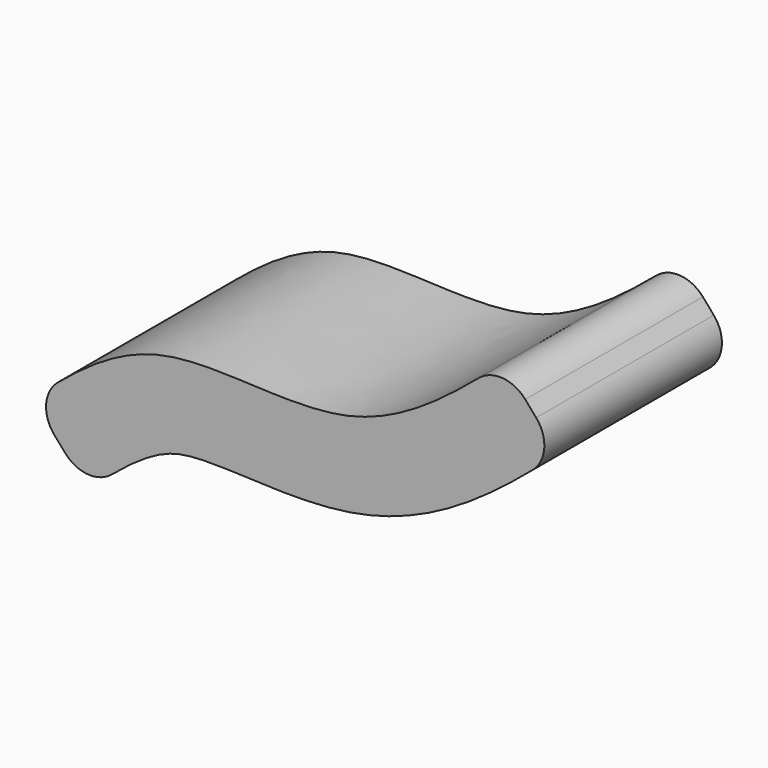
from build123d import *

# Parameters (mm, degrees)
F1_DEPTH = 50.8
F2_R     = 7.62


# Not quite as in the source:
# - the dataset's text gives a spline's control points without its knots; the knots are read off the source's solid


with BuildPart() as f1:
    # F0 (on Front) → F1 (new body)
    with BuildSketch(Plane.XZ):
        with BuildLine():
            add(Edge.make_bspline(
                [(-46.1671091616, 0), (-37.1033304025, 7.9272261416), (-18.0786162948, 24.5663360559), (28.0755181864, 12.987372443), (50.4588119298, 32.4166765689), (61.6594180465, 42.1391054988)],
                knots=[0, 0, 0, 0, 0.3125267415, 0.6559881994, 1, 1, 1, 1], degree=3))
            Line((-46.1671091616, 0), (-33.6258047307, -14.3393927058))
            add(Edge.make_bspline(
                [(-33.6258047307, -14.3393927058), (-31.8132040881, -12.7540831368), (-29.2307453089, -10.4982277646), (-26.0239095445, -7.8573374421), (-23.7368914894, -6.0858011695), (-21.5707475447, -4.5442227641), (-19.5307469779, -3.245218017), (-17.9388050177, -2.3665345235), (-16.727470375, -1.7805087063), (-15.8478404371, -1.3968942034), (-14.9938941443, -1.0662973184), (-14.1605211756, -0.7853779615), (-13.4786898496, -0.5901216464), (-12.9347342127, -0.4553712905), (-12.5313477685, -0.3657981044), (-12.1108276326, -0.2832227824), (-11.499360182, -0.1779155125), (-10.6531211267, -0.0601801028), (-9.506378484, 0.0540683405), (-7.8116614744, 0.1655444659), (-5.3990680173, 0.2238787266), (-2.0914286493, 0.1737882575), (1.5768937561, 0.036826116), (5.5655375148, -0.1377780767), (9.8466834942, -0.2876796945), (14.4042409141, -0.3378589812), (18.4267567915, -0.2219353613), (21.7774575995, 0.0200764532), (24.3553536476, 0.2921382449), (26.5567209981, 0.6087258627), (28.3456316483, 0.9247611681), (29.7056002144, 1.1967067305), (31.061914682, 1.5015091652), (32.8423524074, 1.9452744823), (35.0245121355, 2.569138395), (37.5677349315, 3.417523471), (40.8577819604, 4.6683606746), (44.7801597612, 6.4309792423), (49.1954474176, 8.7903112069), (54.7257632475, 12.176709092), (61.0427228557, 16.7216035375), (67.9007363739, 22.3290908204), (72.1120930692, 25.9865496503), (74.1470171068, 27.7529187313)],
                knots=[0, 0, 0, 0, 0.0625, 0.09375, 0.125, 0.15625, 0.1875, 0.21875, 0.234375, 0.25, 0.265625, 0.28125, 0.296875, 0.3046875, 0.3125, 0.3203125, 0.328125, 0.34375, 0.359375, 0.375, 0.40625, 0.4375, 0.46875, 0.5, 0.53125, 0.5625, 0.59375, 0.609375, 0.625, 0.640625, 0.6484375, 0.65625, 0.6640625, 0.671875, 0.6875, 0.703125, 0.71875, 0.75, 0.78125, 0.8125, 0.875, 0.9375, 1, 1, 1, 1], degree=3))
            Line((74.1470171068, 27.7529187313), (61.6594180465, 42.1391054988))
        make_face()
    extrude(amount=F1_DEPTH)

    # F2
    f2_edges = [f1.edges().sort_by_distance(p)[0] for p in [
        (61.659418, -25.4, 42.139105),
        (74.147017, -25.4, 27.752919),
        (-46.167109, -25.4, 0),
        (-33.625805, -25.4, -14.339393),
    ]]
    fillet(f2_edges, radius=F2_R)


solid = f1.part
